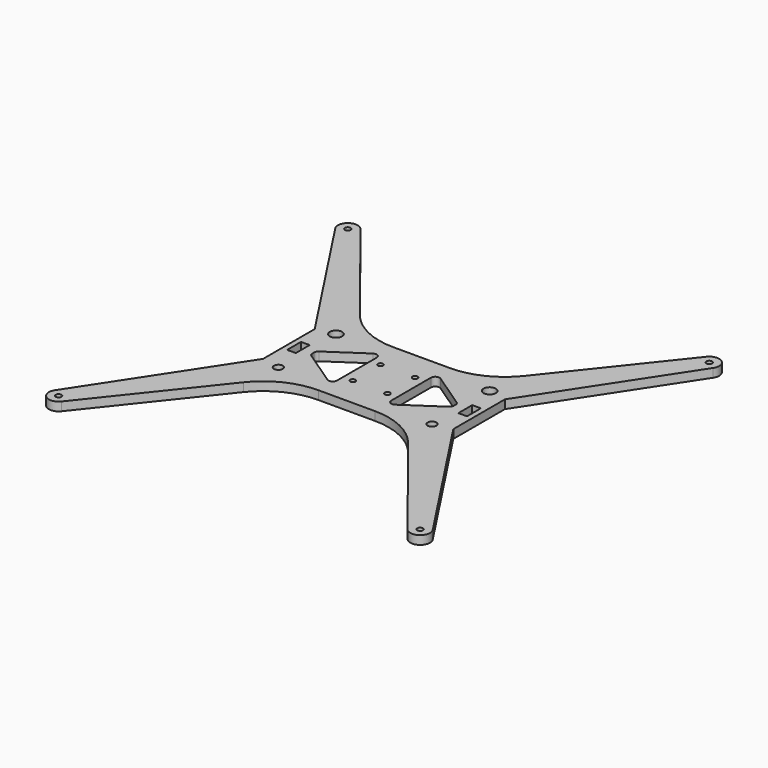
from build123d import *

# Parameters (mm, degrees)
F0_R     = 1.65
F0_R_2   = 2.55
F0_W     = 5
F0_H     = 10
F0_R_3   = 1.5
F0_R_4   = 3.555
F1_DEPTH = 5


# Not quite as in the source:
# - ends of sketch curves that miss each other by under 0.0002 mm in the source are joined


with BuildPart() as f1:
    # F0 (on Top) → F1 (new body)
    with BuildSketch(Plane.XY):
        with BuildLine():
            Line((-47.640397, 42.115595), (-100.031737, 108.050449))
            ThreePointArc((-100.031737, 108.050449), (-107.8442155419, 109.1246397394), (-109.2715048598, 101.368896092))
            Line((-109.2715048598, 101.368896092), (-54.999977, 18.664241))
            Line((-54.999977, 18.664241), (-54.999977, -18.664242))
            Line((-54.999977, -18.664242), (-109.271505, -101.368897))
            ThreePointArc((-109.271505, -101.368897), (-107.8441644553, -109.1246766812), (-100.031658534, -108.0503513703))
            Line((-100.031658534, -108.0503513703), (-47.643302, -42.116283))
            ThreePointArc((-47.643302, -42.116283), (-33.7130803066, -30.9767526972), (-16.325566, -27))
            Line((-16.325566, -27), (16.325565, -27))
            ThreePointArc((16.325565, -27), (33.7130793066, -30.9767526972), (47.6433013924, -42.1162826882))
            Line((47.6433013924, -42.1162826882), (100.031658, -108.050351))
            ThreePointArc((100.031658, -108.050351), (107.8441644255, -109.1246767027), (109.2715050175, -101.3688963323))
            Line((109.2715050175, -101.3688963323), (54.999976, -18.664242))
            Line((54.999976, -18.664242), (54.999976, 18.664241))
            Line((54.999976, 18.664241), (109.271504, 101.368896))
            ThreePointArc((109.271504, 101.368896), (107.8442155121, 109.1246397609), (100.0317360662, 108.0504489474))
            Line((100.0317360662, 108.0504489474), (47.640396, 42.115595))
            ThreePointArc((47.640396, 42.115595), (33.7103248028, 30.9765618002), (16.323206, 27))
            Line((16.323206, 27), (-16.323206, 27))
            ThreePointArc((-16.323206, 27), (-33.710325083, 30.9765619354), (-47.640397, 42.115595))
        make_face()
        with Locations((-104.5, -104.5)):
            Circle(F0_R, mode=Mode.SUBTRACT)
        with Locations((-44.444977, -20.807752)):
            Circle(F0_R_2, mode=Mode.SUBTRACT)
        with Locations((-49.499977, 0)):
            Rectangle(F0_W, F0_H, mode=Mode.SUBTRACT)
        with BuildLine():
            Line((-19.581953, -16.373154), (-39.803759, -2.743263))
            ThreePointArc((-39.803759, -2.743263), (-40.6136447533, -1.8442487652), (-40.906473, -0.670199))
            Line((-40.906473, -0.670199), (-40.906473, 0.670176))
            ThreePointArc((-40.906473, 0.670176), (-40.6136450793, 1.8442251525), (-39.8037598701, 2.7432388072))
            Line((-39.8037598701, 2.7432388072), (-19.581955, 16.373149))
            ThreePointArc((-19.581955, 16.373149), (-17.0106188475, 16.5072580793), (-15.684668, 14.300086))
            Line((-15.684668, 14.300086), (-15.684668, -14.30009))
            ThreePointArc((-15.684668, -14.30009), (-17.0106178687, -16.5072615586), (-19.581953, -16.373154))
        make_face(mode=Mode.SUBTRACT)
        with Locations((-10, -10)):
            Circle(F0_R_3, mode=Mode.SUBTRACT)
        with Locations((104.5, -104.5)):
            Circle(F0_R, mode=Mode.SUBTRACT)
        with Locations((10, -10)):
            Circle(F0_R_3, mode=Mode.SUBTRACT)
        with Locations((44.444976, -20.807752)):
            Circle(F0_R_2, mode=Mode.SUBTRACT)
        with BuildLine():
            Line((19.581954, 16.373149), (39.803759, 2.743239))
            ThreePointArc((39.803759, 2.743239), (40.6136440793, 1.8442251525), (40.906472, 0.670176))
            Line((40.906472, 0.670176), (40.906472, -0.670199))
            ThreePointArc((40.906472, -0.670199), (40.6136437533, -1.8442487652), (39.803757719, -2.7432625831))
            Line((39.803757719, -2.7432625831), (19.581952, -16.373154))
            ThreePointArc((19.581952, -16.373154), (17.0106168687, -16.5072615586), (15.684667, -14.30009))
            Line((15.684667, -14.30009), (15.684667, 14.300086))
            ThreePointArc((15.684667, 14.300086), (17.0106178475, 16.5072580793), (19.581954, 16.373149))
        make_face(mode=Mode.SUBTRACT)
        with Locations((49.499976, 0)):
            Rectangle(F0_W, F0_H, mode=Mode.SUBTRACT)
        with Locations((-44.444977, 20.810818)):
            Circle(F0_R_4, mode=Mode.SUBTRACT)
        with Locations((-10, 10)):
            Circle(F0_R_3, mode=Mode.SUBTRACT)
        with Locations((-104.5, 104.5)):
            Circle(F0_R, mode=Mode.SUBTRACT)
        with Locations((10, 10)):
            Circle(F0_R_3, mode=Mode.SUBTRACT)
        with Locations((44.444976, 20.810818)):
            Circle(F0_R_4, mode=Mode.SUBTRACT)
        with Locations((104.5, 104.5)):
            Circle(F0_R, mode=Mode.SUBTRACT)
    extrude(amount=F1_DEPTH)


solid = f1.part
